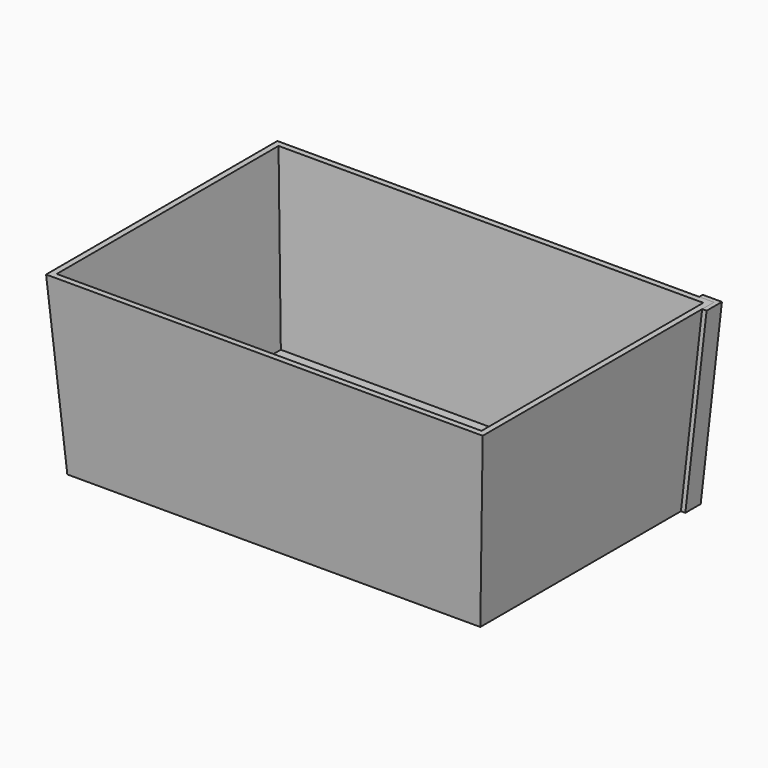
from build123d import *

# Parameters (mm, degrees)
F0_W        = 150
F0_H        = 100
F1_DEPTH    = 60
F2_T1_DEPTH = 539.968053853
F2_T3_DEPTH = 489.968053853
F3_T        = -2


# Not quite as in the source:
# - a fillet or chamfer that OpenCascade refuses, or shapes differently, is made with other operations: its cross-section is extruded or revolved along the edge and cut away or added


with BuildPart() as f1:
    # F0 (on Top) → F1 (new body)
    with BuildSketch(Plane.XY):
        Rectangle(F0_W, F0_H)
    extrude(amount=F1_DEPTH)

    # F2: chamfer of 5 x 75 on 4 edges, made by hand

    # F2_s2 → F2_t1 (cut)
    with BuildSketch(Plane.YZ.offset(-269.9840269265)):
        Polygon((-50, 75), (-45, 0), (-50, 0), align=None)
        Polygon((50, 75), (45, 0), (50, 0), align=None)
    extrude(amount=F2_T1_DEPTH, mode=Mode.SUBTRACT)

    # F2_s4 → F2_t3 (cut)
    with BuildSketch(Plane.XZ.offset(-244.9840269265)):
        Polygon((75, 75), (70, 0), (75, 0), align=None)
        Polygon((-75, 75), (-70, 0), (-75, 0), align=None)
    extrude(amount=F2_T3_DEPTH, mode=Mode.SUBTRACT)

    # F3
    f3_openings = [f1.faces().sort_by_distance(p)[0] for p in [
        (0, 0, 60),
    ]]
    offset(amount=F3_T, openings=f3_openings)


with BuildPart() as f5:
    # F5: sweep along a path in F5_path
    with BuildLine(Plane(origin=(70, 45, 0), x_dir=(0, -0.0665190105, -0.9977851579), z_dir=(0, 0.9977851579, -0.0665190105))) as f5_path:
        Line((0, 0), (-60.1331855135, -4))
    # F4 (on face) → F5 (sweep)
    with BuildSketch(Plane.XY.offset(60)):
        Polygon((69, 49), (74, 49), (74, 44), (75.5, 44), (75.5, 50.5), (69, 50.5), align=None)
    sweep(path=f5_path.line)


solid = Compound([f1.part, f5.part])
